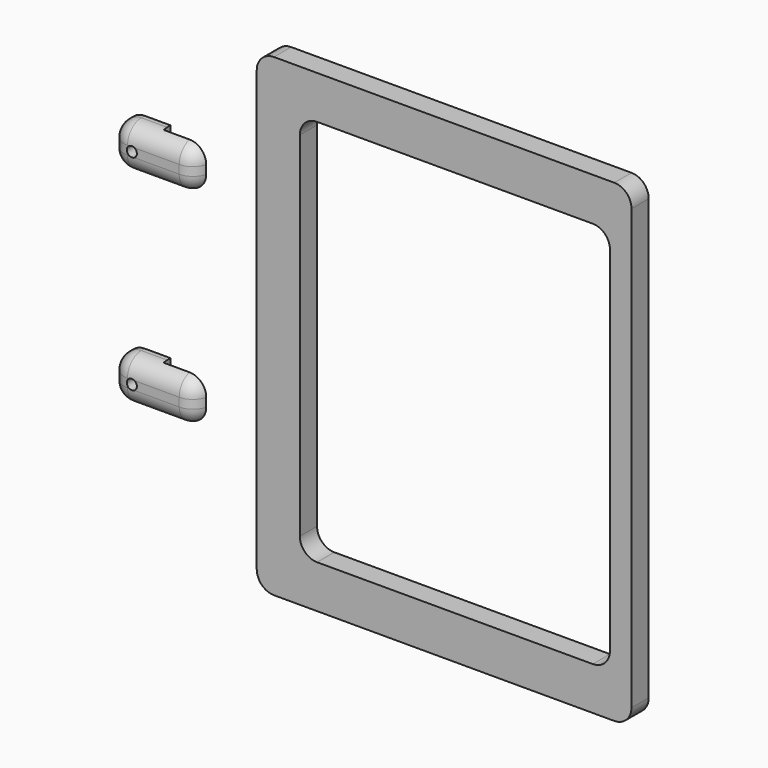
from build123d import *

# Parameters (mm, degrees)
F0_W     = 110.49
F0_H     = 139.7
F0_W_2   = 91.44
F0_H_2   = 114.3
F2_DEPTH = 6.35
F3_R     = 5.08
F1_W     = 0.0457762241
F1_H     = 12.7
F1_W_2   = 12.6542237759
F4_DEPTH = 6.35
F1_W_3   = 12.7
F1_H_2   = 12.6999970629
F5_R     = 5.08
F6_R     = 5.08
F7_W     = 12.7
F7_H     = 15.24
F8_DEPTH = 2.54
F9_DEPTH = 2.54
F11_D    = 2.9718
F12_D    = 2.9718


# Not quite as in the source:
# - a feature of the source that left no trace in its solid (it failed there, or was rolled back) is left out


with BuildPart() as f2:
    # F0 (on Front) → F2 (new body)
    with BuildSketch(Plane.XZ):
        with Locations((-3.175, 0)):
            Rectangle(F0_W, F0_H)
        Rectangle(F0_W_2, F0_H_2, mode=Mode.SUBTRACT)
    extrude(amount=F2_DEPTH)

    # F3
    f3_edges = [f2.edges().sort_by_distance(p)[0] for p in [
        (-58.42, -3.175, 69.85),
        (-58.42, -3.175, -69.85),
        (52.07, -3.175, -69.85),
        (52.07, -3.175, 69.85),
        (-45.72, -3.175, 57.15),
        (45.72, -3.175, 57.15),
        (45.72, -3.175, -57.15),
        (-45.72, -3.175, -57.15),
    ]]
    fillet(f3_edges, radius=F3_R)


with BuildPart() as f4:
    # F1 (on Front) → F4 (new body)
    with BuildSketch(Plane.XZ):
        with Locations((-76.2228881121, 31.618843414)):
            Rectangle(F1_W, F1_H)
        with Locations((-82.5728881121, 31.618843414)):
            Rectangle(F1_W_2, F1_H)
        with Locations((-88.9228881121, 31.618843414)):
            Rectangle(F1_W, F1_H)
        with Locations((-95.2728881121, 31.618843414)):
            Rectangle(F1_W_2, F1_H)
    extrude(amount=F4_DEPTH)

    # F5
    f5_edges = [f4.edges().sort_by_distance(p)[0] for p in [
        (-101.6, -3.175, 37.968843),
        (-88.9, -6.35, 37.968843),
        (-76.2, -6.35, 31.618843),
        (-88.9, -6.35, 25.268843),
        (-76.2, -3.175, 25.268843),
        (-101.6, -3.175, 25.268843),
        (-76.2, -3.175, 37.968843),
        (-101.6, -6.35, 31.618843),
    ]]
    fillet(f5_edges, radius=F5_R)

    # F7 (on Front) → F8 (cut)
    with BuildSketch(Plane.XZ):
        with Locations((-82.55, 31.543379275)):
            Rectangle(F7_W, F7_H)
    extrude(amount=F8_DEPTH, mode=Mode.SUBTRACT)

    # F11 (through all)
    with Locations(Plane(origin=(0, 0, 0), x_dir=(1, 0, 0), z_dir=(0, 1, 0))):
        with Locations((-95.25, -31.618843414)):
            Hole(F11_D / 2)


with BuildPart() as f4b:
    # F1 (on Front) → F4, piece 2 (new body)
    with BuildSketch(Plane.XZ):
        with Locations((-82.55, -28.8023503282)):
            Rectangle(F1_W_3, F1_H_2)
        with Locations((-95.25, -28.8023503282)):
            Rectangle(F1_W_3, F1_H_2)
    extrude(amount=F4_DEPTH)

    # F6
    f6_edges = [f4b.edges().sort_by_distance(p)[0] for p in [
        (-88.9, -6.35, -22.452352),
        (-76.2, -6.35, -28.80235),
        (-101.6, -6.35, -28.80235),
        (-88.9, -6.35, -35.152349),
        (-101.6, -3.175, -35.152349),
        (-101.6, -3.175, -22.452352),
        (-76.2, -3.175, -35.152349),
        (-76.2, -3.175, -22.452352),
    ]]
    fillet(f6_edges, radius=F6_R)

    # F7 (on Front) → F9 (cut)
    with BuildSketch(Plane.XZ):
        with Locations((-82.55, 31.543379275)):
            Rectangle(F7_W, F7_H)
        with Locations((-82.55, -28.520518263)):
            Rectangle(F7_W, F7_H)
    extrude(amount=F9_DEPTH, mode=Mode.SUBTRACT)

    # F12 (through all)
    with Locations(Plane(origin=(0, 0, 0), x_dir=(1, 0, 0), z_dir=(0, 1, 0))):
        with Locations((-95.25, 28.8023517968)):
            Hole(F12_D / 2)


solid = Compound([f2.part, f4.part, f4b.part])
